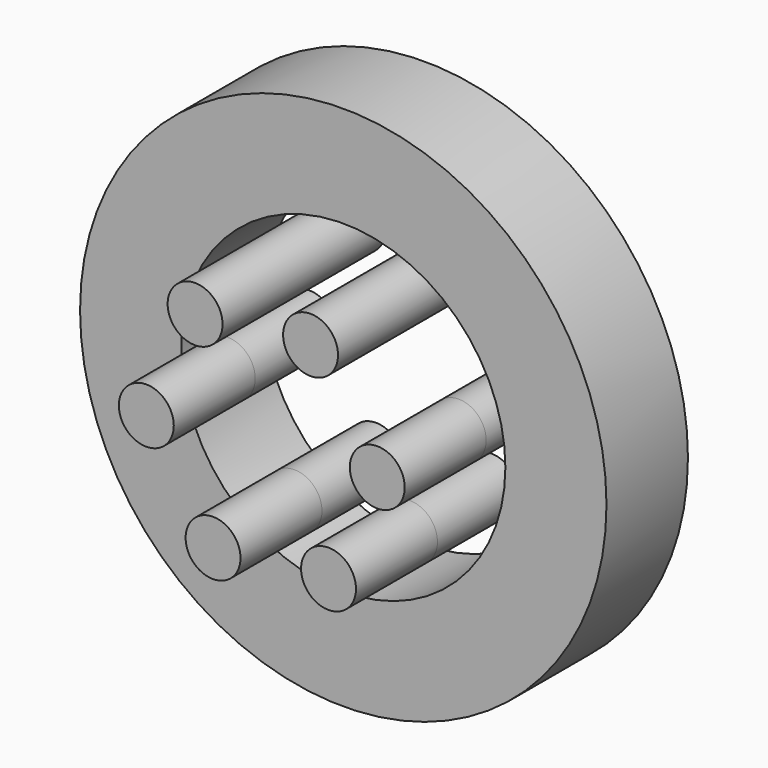
from build123d import *

# Parameters (mm, degrees)
F0_R     = 65.6559309804
F0_R_2   = 40.4354066136
F3_DEPTH = 25.4
F4_R     = 6.847573374
F5_DEPTH = 25.4
F6_DEPTH = 25.4
F7_DEPTH = 25.4
F8_DEPTH = 25.4


# Not quite as in the source:
# - the program builds the solid bodies; features that only make, move or delete a surface that nothing else refers to are left out


with BuildPart() as f3:
    # F0 (on Front) → F3 (new body)
    with BuildSketch(Plane.XZ):
        Circle(F0_R)
        Circle(F0_R_2, mode=Mode.SUBTRACT)
    extrude(amount=F3_DEPTH)


with BuildPart() as f5:
    # F4 (on Front) → F5 (new body)
    with BuildSketch(Plane.XZ):
        with Locations((12.1613769004, 28.0169486328)):
            Circle(F4_R)
    extrude(amount=F5_DEPTH)

    # F8 (add): a face of the model
    f8_faces = [f5.faces().sort_by_distance(p)[0] for p in [
        (12.1613769004, -25.4, 28.0169486328),
    ]]
    extrude(f8_faces, amount=F8_DEPTH)


with BuildPart() as f5b:
    # F4 (on Front) → F5, piece 2 (new body)
    with BuildSketch(Plane.XZ):
        with Locations((-16.6429076344, 25.4295356572)):
            Circle(F4_R)
    extrude(amount=F5_DEPTH)

    # F7 (add): a face of the model
    f7_faces = [f5b.faces().sort_by_distance(p)[0] for p in [
        (-16.6429076344, -25.4, 25.4295356572),
    ]]
    extrude(f7_faces, amount=F7_DEPTH)


with BuildPart() as f5c:
    # F4 (on Front) → F5, piece 3 (new body)
    with BuildSketch(Plane.XZ):
        with Locations((-28.8042845348, -0.8094129756)):
            Circle(F4_R)
    extrude(amount=F5_DEPTH)


with BuildPart() as f5d:
    # F4 (on Front) → F5, piece 4 (new body)
    with BuildSketch(Plane.XZ):
        with Locations((-12.1613769004, -24.4609486328)):
            Circle(F4_R)
    extrude(amount=F5_DEPTH)


with BuildPart() as f5e:
    # F4 (on Front) → F5, piece 5 (new body)
    with BuildSketch(Plane.XZ):
        with Locations((16.6429076344, -21.8735356572)):
            Circle(F4_R)
    extrude(amount=F5_DEPTH)


with BuildPart() as f5f:
    # F4 (on Front) → F5, piece 6 (new body)
    with BuildSketch(Plane.XZ):
        with Locations((28.8042845348, 4.3654129756)):
            Circle(F4_R)
    extrude(amount=F5_DEPTH)


with BuildPart() as f6:
    # F6 (new): a face of the model
    f6_faces = [f5d.part.faces().sort_by_distance(p)[0] for p in [
        (-12.1613769004, -25.4, -24.4609486328),
    ]]
    extrude(f6_faces, amount=F6_DEPTH)


with BuildPart() as f6b:
    # F6#2 (new): a face of the model
    f6_2_faces = [f5e.part.faces().sort_by_distance(p)[0] for p in [
        (16.6429076344, -25.4, -21.8735356572),
    ]]
    extrude(f6_2_faces, amount=F6_DEPTH)


with BuildPart() as f6c:
    # F6#3 (new): a face of the model
    f6_3_faces = [f5f.part.faces().sort_by_distance(p)[0] for p in [
        (28.8042845348, -25.4, 4.3654129756),
    ]]
    extrude(f6_3_faces, amount=F6_DEPTH)


with BuildPart() as f6d:
    # F6#4 (new): a face of the model
    f6_4_faces = [f5c.part.faces().sort_by_distance(p)[0] for p in [
        (-28.8042845348, -25.4, -0.8094129756),
    ]]
    extrude(f6_4_faces, amount=F6_DEPTH)


solid = Compound([f3.part, f5.part, f5b.part, f5c.part, f5d.part, f5e.part, f5f.part, f6.part, f6b.part, f6c.part, f6d.part])
